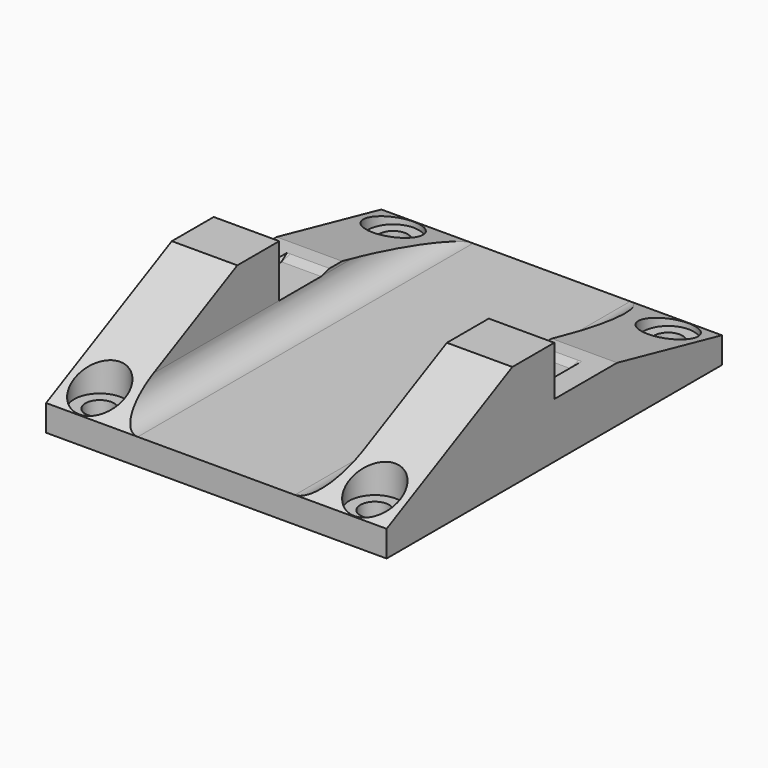
from build123d import *

# Parameters (mm, degrees)
F1_DEPTH       = 32.5
F2_W           = 40
F2_H           = 15
F3_DEPTH       = 40.001
F3_DEPTH_BACK  = 40.001
F4_R           = 4.99999
F6_D           = 5.5
F6_START       = 4.9375
F6_START_2     = 4.9723205
F6_CBORE_D     = 9.75
F6_CBORE_DEPTH = 1
F7_W           = 5
F7_H           = 12
F8_DEPTH       = 0.5358983849
F9_T4_DEPTH    = 13.5430097928
F9_T10_DEPTH   = 13.5430097928


# Not quite as in the source:
# - a fillet or chamfer that OpenCascade refuses, or shapes differently, is made with other operations: its cross-section is extruded or revolved along the edge and cut away or added
# - a fillet or chamfer is up to 0.001 mm smaller than in the source, because OpenCascade refuses the exact size


with BuildPart() as f1:
    # F0 (on Right) → F1 (new body, symmetric)
    with BuildSketch(Plane.YZ):
        Polygon((0, 10), (0, 20), (-10, 20), (-40, 5), (-40, 0), (40, 0), (40, 5), (15, 10.5358983849), (12, 10.5358983849), (10, 10), align=None)
    extrude(amount=F1_DEPTH, both=True)

    # F2 (on Front) → F3 (cut, two sides)
    with BuildSketch(Plane.XZ) as f3_sk:
        with Locations((0, 12.5)):
            Rectangle(F2_W, F2_H)
    extrude(amount=-F3_DEPTH, mode=Mode.SUBTRACT)
    extrude(f3_sk.sketch, amount=F3_DEPTH_BACK, mode=Mode.SUBTRACT)

    # F4 (radius 5 in the source; OpenCascade refuses exactly that, so slightly less here)
    f4_edges = [f1.edges().sort_by_distance(p)[0] for p in [
        (20, 0, 5),
        (-20, 0, 5),
    ]]
    fillet(f4_edges, radius=F4_R)

    # F6 (through all)
    # its depths count from where the whole tool has entered the part; down to there all is cleared
    with Locations(Plane.XY.offset(10)):
        with Locations((-26.25, 35, -F6_START_2), (26.25, 35, -F6_START_2), (-26.25, -35, -F6_START), (26.25, -35, -F6_START)):
            CounterBoreHole(F6_D / 2, F6_CBORE_D / 2, F6_CBORE_DEPTH)

    # F7 (on face) → F8 (join, through all)
    with BuildSketch(Plane.XY.offset(10)):
        with Locations((-30, 6)):
            Rectangle(F7_W, F7_H)
        with Locations((30, 6)):
            Rectangle(F7_W, F7_H)
    extrude(amount=F8_DEPTH)

    # F9: chamfer of 0.6 on 2 edges, made by hand


with BuildPart() as f9_tool2:
    # F9_s3 → F9_t4 (new body)
    with BuildSketch(Plane.XZ.offset(-13.5430097928)):
        Polygon((27.5, 9.9358983849), (28.1, 10.5358983849), (27.5, 10.5358983849), align=None)
    extrude(amount=F9_T4_DEPTH)

    split(bisect_by=Plane(origin=(0, -1.8301270189, 6.8301270189), x_dir=(1, 0, 0), z_dir=(0, -0.2588190451, 0.9659258263)), keep=Keep.TOP)

    split(bisect_by=Plane.XY.offset(10), keep=Keep.TOP)


with BuildPart() as f1_1:
    add(f1.part)

    # F9_t1: cut F9_tool2
    add(f9_tool2.part, mode=Mode.SUBTRACT)


with BuildPart() as f9_tool8:
    # F9_s9 → F9_t10 (new body)
    with BuildSketch(Plane.XZ):
        Polygon((-27.5, 9.9358983849), (-28.1, 10.5358983849), (-27.5, 10.5358983849), align=None)
    extrude(amount=-F9_T10_DEPTH)

    split(bisect_by=Plane(origin=(0, -1.8301270189, 6.8301270189), x_dir=(1, 0, 0), z_dir=(0, -0.2588190451, 0.9659258263)), keep=Keep.TOP)

    split(bisect_by=Plane.XY.offset(10), keep=Keep.TOP)


with BuildPart() as f1_2:
    add(f1_1.part)

    # F9_t7: cut F9_tool8
    add(f9_tool8.part, mode=Mode.SUBTRACT)


solid = f1_2.part
